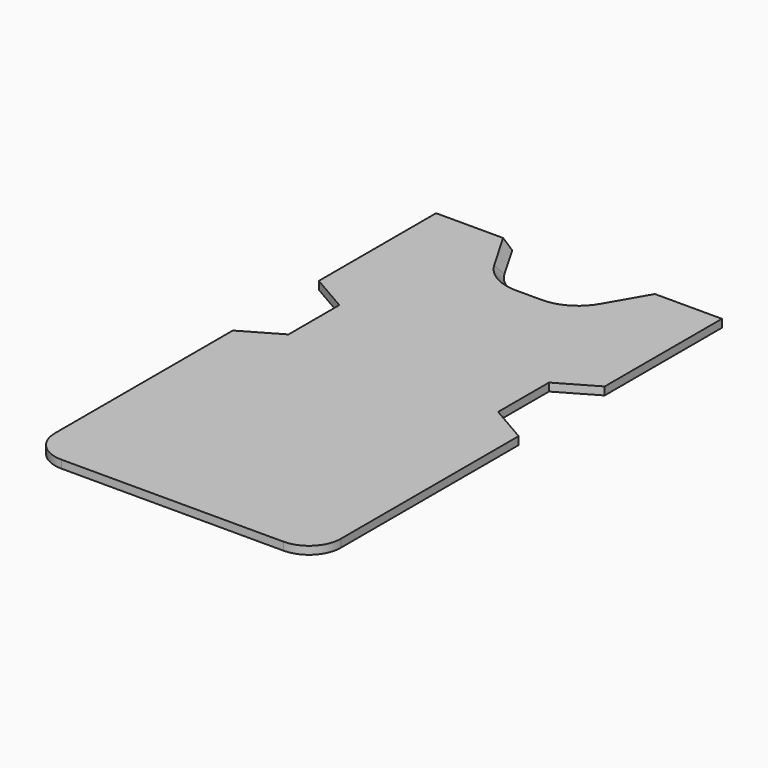
from build123d import *

# Parameters (mm, degrees)
F0_W     = 114.3
F0_H     = 50.8
F1_DEPTH = 3.175
F2_DEPTH = 152.4
F4_DEPTH = 3.302
F5_R     = 15.24
F6_R     = 12.7
F7_DEPTH = 3.175
F8_SIZE  = 3.17499


# Not quite as in the source:
# - a fillet or chamfer is up to 0.001 mm smaller than in the source, because OpenCascade refuses the exact size


with BuildPart() as f1:
    # F0 (on Top) → F1 (new body)
    with BuildSketch(Plane.XY):
        Rectangle(F0_W, F0_H)
    extrude(amount=F1_DEPTH)

    # F2 (add): a face of the model
    f2_faces = [f1.faces().sort_by_distance(p)[0] for p in [
        (0, 25.4, 1.5875),
    ]]
    extrude(f2_faces, amount=F2_DEPTH)

    # F3 (on face) → F4 (cut)
    with BuildSketch(Plane.XY.offset(3.175)):
        Polygon((-13.97, 155.8029547439), (13.97, 155.8029547439), (26.67, 177.8), (-26.67, 177.8), align=None)
    extrude(amount=-F4_DEPTH, mode=Mode.SUBTRACT)

    # F5
    f5_edges = [f1.edges().sort_by_distance(p)[0] for p in [
        (13.97, 155.802955, 1.5875),
        (-13.97, 155.802955, 1.5875),
    ]]
    fillet(f5_edges, radius=F5_R)

    # F6
    f6_edges = [f1.edges().sort_by_distance(p)[0] for p in [
        (57.15, -25.4, 1.5875),
        (-57.15, -25.4, 1.5875),
    ]]
    fillet(f6_edges, radius=F6_R)

    # F3 (on face) → F7 (cut)
    with BuildSketch(Plane.XY.offset(3.175)):
        Polygon((57.15, 76.2), (57.15, 119.1976362049), (41.91, 110.3988181024), (41.91, 84.9988181024), align=None)
        Polygon((-41.91, 110.3988181024), (-57.15, 119.1976362049), (-57.15, 76.2), (-41.91, 84.9988181024), align=None)
    extrude(amount=-F7_DEPTH, mode=Mode.SUBTRACT)

    # F8 (size 3.175 in the source; OpenCascade refuses exactly that, so slightly less here)
    f8_edges = [f1.edges().sort_by_distance(p)[0] for p in [
        (-22.519705, 170.611477, 3.175),
        (-12.791182, 157.844728, 3.175),
        (0, 155.802955, 3.175),
        (12.791182, 157.844728, 3.175),
        (22.519705, 170.611477, 3.175),
    ]]
    chamfer(f8_edges, length=F8_SIZE)


solid = f1.part
